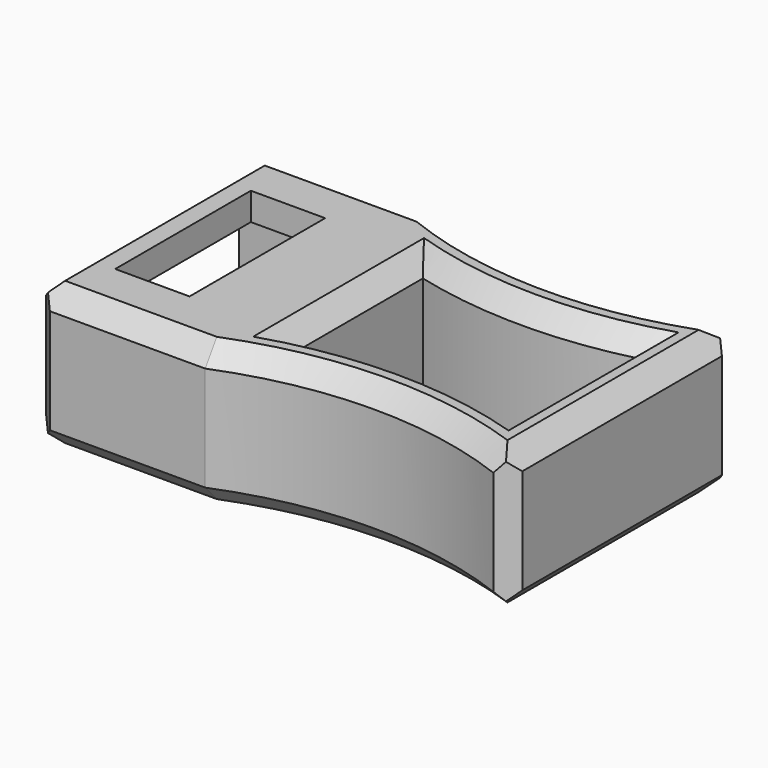
from build123d import *

# Parameters (mm, degrees)
F0_W         = 25
F0_H         = 15.1
F1_DEPTH     = 7.5
F2_W         = 12.2
F2_H         = 4.6
F3_DEPTH     = 9.95
F4_W         = 3.9
F4_H         = 8.9
F5_DEPTH     = 25
F6_SIZE      = 1
F7_C1_SIZE   = 1
F7_C2_SIZE   = 1
F7_C3_SIZE   = 1
F7_C4_SIZE   = 1
F7_C5_SIZE   = 1
F7_C6_SIZE   = 1
F7_C7_SIZE   = 1
F7_C8_SIZE   = 1
F8_R         = 20.5
F9_DEPTH     = 25
F10_T2_ANGLE = 49.7995158882
F10_T4_ANGLE = 49.7995158882
F10_T6_ANGLE = 49.7995158882
F10_T8_ANGLE = 49.7995158882
F12_DEPTH    = 25
F13_SIZE     = 1
F14_W        = 6.9057337241
F14_H        = 9.9417776801
F15_DEPTH    = 0.5


# Not quite as in the source:
# - a fillet or chamfer that OpenCascade refuses, or shapes differently, is made with other operations: its cross-section is extruded or revolved along the edge and cut away or added


with BuildPart() as f1:
    # F0 (on Top) → F1 (new body)
    with BuildSketch(Plane.XY):
        with Locations((12.5, 0)):
            Rectangle(F0_W, F0_H)
    extrude(amount=F1_DEPTH)

    # F2 (on face) → F3 (cut)
    with BuildSketch(Plane(origin=(0, 0, 0), x_dir=(0, -1, 0), z_dir=(-1, 0, 0))):
        with Locations((0, 3.75)):
            Rectangle(F2_W, F2_H)
    extrude(amount=-F3_DEPTH, mode=Mode.SUBTRACT)

    # F4 (on face) → F5 (cut)
    with BuildSketch(Plane.XY.offset(7.5)):
        with Locations((3.9, 0)):
            Rectangle(F4_W, F4_H)
    extrude(amount=-F5_DEPTH, mode=Mode.SUBTRACT)

    # F6
    f6_edges = [f1.edges().sort_by_distance(p)[0] for p in [
        (25, -7.55, 3.75),
        (25, 7.55, 3.75),
        (25, 0, 0),
        (25, 0, 7.5),
    ]]
    chamfer(f6_edges, length=F6_SIZE)

    # F7: chamfer of 1 on 8 edges, made by hand

    # F7_c1
    f7_c1_edges = [f1.edges().sort_by_distance(p)[0] for p in [
        (12, -7.55, 0),
    ]]
    chamfer(f7_c1_edges, length=F7_C1_SIZE)

    # F7_c2
    f7_c2_edges = [f1.edges().sort_by_distance(p)[0] for p in [
        (0, -7.55, 4.25),
    ]]
    chamfer(f7_c2_edges, length=F7_C2_SIZE)

    # F7_c3
    f7_c3_edges = [f1.edges().sort_by_distance(p)[0] for p in [
        (12.5, -7.55, 7.5),
    ]]
    chamfer(f7_c3_edges, length=F7_C3_SIZE)

    # F7_c4
    f7_c4_edges = [f1.edges().sort_by_distance(p)[0] for p in [
        (0, 0.5, 0),
    ]]
    chamfer(f7_c4_edges, length=F7_C4_SIZE)

    # F7_c5
    f7_c5_edges = [f1.edges().sort_by_distance(p)[0] for p in [
        (12.5, 7.55, 0),
    ]]
    chamfer(f7_c5_edges, length=F7_C5_SIZE)

    # F7_c6
    f7_c6_edges = [f1.edges().sort_by_distance(p)[0] for p in [
        (0, 0.5, 7.5),
    ]]
    chamfer(f7_c6_edges, length=F7_C6_SIZE)

    # F7_c7
    f7_c7_edges = [f1.edges().sort_by_distance(p)[0] for p in [
        (12.5, 7.55, 7.5),
    ]]
    chamfer(f7_c7_edges, length=F7_C7_SIZE)

    # F7_c8
    f7_c8_edges = [f1.edges().sort_by_distance(p)[0] for p in [
        (0, 7.55, 3.75),
    ]]
    chamfer(f7_c8_edges, length=F7_C8_SIZE)

    # F8 (on face) → F9 (cut)
    with BuildSketch(Plane.XY.offset(7.5)):
        with Locations((16.8532188982, 26.55)):
            Circle(F8_R)
        with Locations((16.8532188982, -26.55)):
            Circle(F8_R)
    extrude(amount=-F9_DEPTH, mode=Mode.SUBTRACT)

    # F10: chamfer of 1 on 4 edges, made by hand

    # F10_s1 → F10_t2 (revolve, cut)
    with BuildSketch(Plane(origin=(24.005003563, -11.1426284002, 0), x_dir=(0, 0, 1), z_dir=(0.907045793, -0.4210319814, 0))):
        Polygon((7.5, -4.5136783409), (6.5, -3.5136783409), (7.5, -3.5136783409), align=None)
    revolve(axis=Axis((16.8532188982, -26.55, 7.5), (0, 0, 1)), revolution_arc=F10_T2_ANGLE, mode=Mode.SUBTRACT)

    # F10_s3 → F10_t4 (revolve, cut)
    with BuildSketch(Plane(origin=(3.7263637991, -1.7297013511, 0), x_dir=(0, 0, 1), z_dir=(-0.907045793, 0.4210319814, 0))):
        Polygon((7.5, 9.6778099504), (6.5, 10.6778099504), (7.5, 10.6778099504), align=None)
    revolve(axis=Axis((16.8532188982, 26.55, 7.5), (0, 0, 1)), revolution_arc=F10_T4_ANGLE, mode=Mode.SUBTRACT)

    # F10_s5 → F10_t6 (revolve, cut)
    with BuildSketch(Plane(origin=(24.005003563, -11.1426284002, 0), x_dir=(0, 0, 1), z_dir=(0.907045793, -0.4210319814, 0))):
        Polygon((1, -3.5136783409), (0, -4.5136783409), (0, -3.5136783409), align=None)
    revolve(axis=Axis((16.8532188982, -26.55, 0), (0, 0, 1)), revolution_arc=F10_T6_ANGLE, mode=Mode.SUBTRACT)

    # F10_s7 → F10_t8 (revolve, cut)
    with BuildSketch(Plane(origin=(3.7263637991, -1.7297013511, 0), x_dir=(0, 0, 1), z_dir=(-0.907045793, 0.4210319814, 0))):
        Polygon((1, 10.6778099504), (0, 9.6778099504), (0, 10.6778099504), align=None)
    revolve(axis=Axis((16.8532188982, 26.55, 0), (0, 0, 1)), revolution_arc=F10_T8_ANGLE, mode=Mode.SUBTRACT)

    # F11 (on face) → F12 (cut)
    with BuildSketch(Plane.XY.offset(7.5)):
        with BuildLine():
            ThreePointArc((11.1193139957, -4.2761962258), (16.8082592809, -3.5500439428), (22.5, -4.2539496056))
            Line((22.5, -4.2539496056), (22.5, 4.2539496056))
            ThreePointArc((22.5, 4.2539496056), (16.8082592809, 3.5500439428), (11.1193139957, 4.2761962258))
            Line((11.1193139957, 4.2761962258), (11.1193139957, -4.2761962258))
        make_face()
    extrude(amount=-F12_DEPTH, mode=Mode.SUBTRACT)

    # F13
    f13_edges = [f1.edges().sort_by_distance(p)[0] for p in [
        (11.119314, 0, 7.5),
        (16.808259, 3.550044, 7.5),
        (22.5, 0, 7.5),
        (16.808259, -3.550044, 7.5),
        (11.119314, 0, 0),
        (16.808259, 3.550044, 0),
        (22.5, 0, 0),
        (16.808259, -3.550044, 0),
    ]]
    chamfer(f13_edges, length=F13_SIZE)

    # F14 (on face) → F15 (join)
    with BuildSketch(Plane(origin=(0, 0, 0), x_dir=(1, 0, 0), z_dir=(0, 0, -1))):
        with Locations((4.9177300534, -0.0320777763)):
            Rectangle(F14_W, F14_H)
    extrude(amount=-F15_DEPTH)


solid = f1.part
